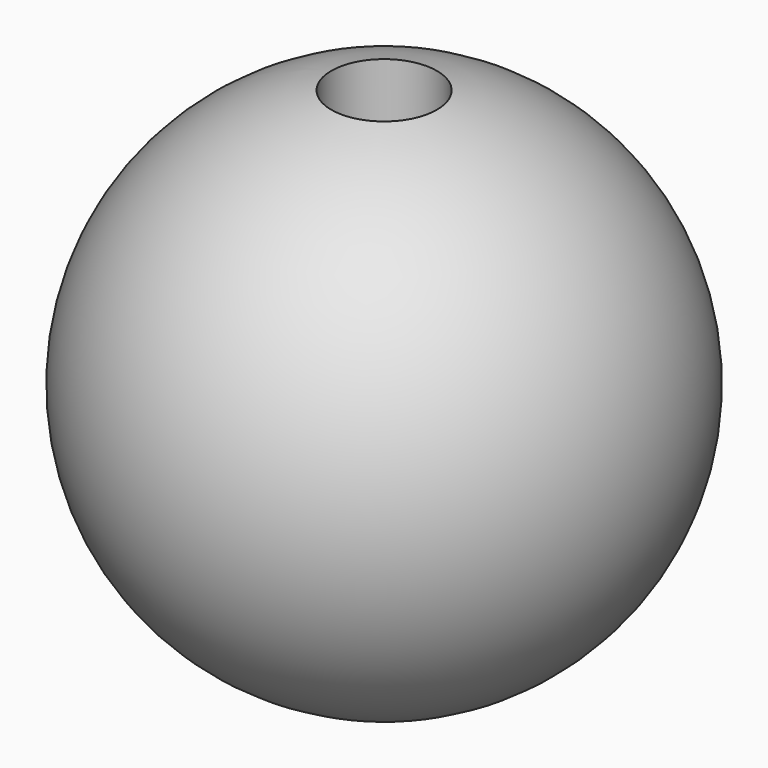
from build123d import *

# Parameters (mm, degrees)
F5_R     = 3.175
F6_DEPTH = 50.8


# Not quite as in the source:
# - a length typed as a fraction of an inch, garbled in the dataset ("3 / 203.2 mm" for 3/8 in), is restored


with BuildPart() as f2:
    # F0 (on Front) → F2 (revolve)
    with BuildSketch(Plane.XZ):
        with BuildLine():
            Line((0, -15.875), (0, 15.875))
            ThreePointArc((0, 15.875), (-15.875, 0), (0, -15.875))
        make_face()
    revolve(axis=Axis((0, 0, 0), (0, 0, 1)))


with BuildPart() as f6:
    # F5 (on offset) → F6 (new body)
    with BuildSketch(Plane.XY.offset(5.715)):
        Circle(F5_R)
    extrude(amount=F6_DEPTH)


with BuildPart() as f2_1:
    add(f2.part)

    # F7: cut F6
    add(f6.part, mode=Mode.SUBTRACT)


solid = f2_1.part
